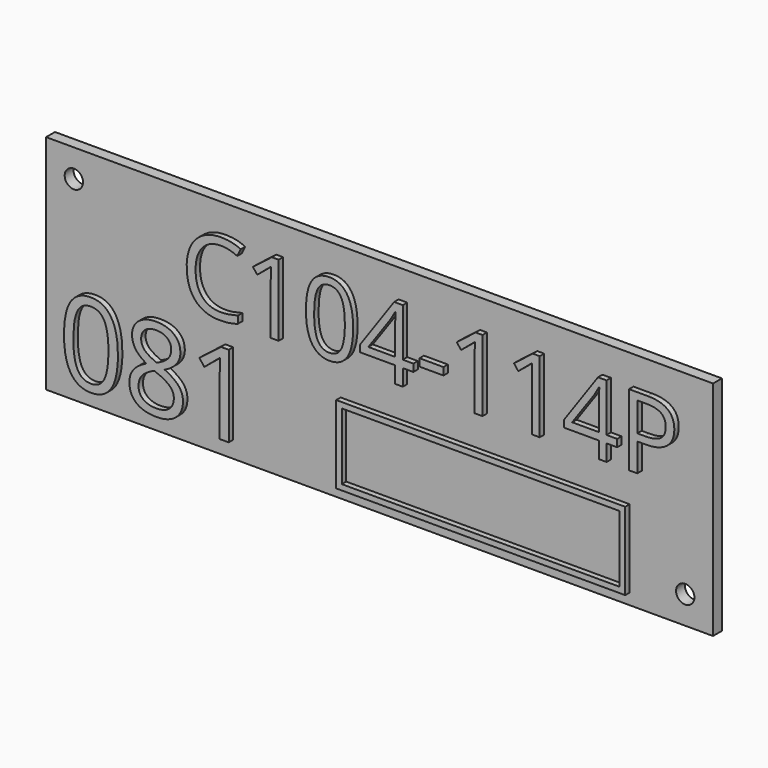
from build123d import *

# Parameters (mm, degrees)
F0_W         = 120
F0_H         = 40
F1_DEPTH     = 2
F3_D         = 3.3
F4_TEXT_SIZE = 18.0050639242
F5_DEPTH     = 1
F6_TEXT_SIZE = 20.5478077656
F7_DEPTH     = 1
F8_W         = 52
F8_H         = 14
F8_W_2       = 49.99999962
F8_H_2       = 11.99999962
F9_DEPTH     = 1


# Not quite as in the source:
# - Text() gives the source's letters only with a copy of the font that has no kerning and outlines rounded to 1/6400 em; it was checked with that copy


with BuildPart() as f1:
    # F0 (on Front) → F1 (new body)
    with BuildSketch(Plane.XZ):
        Rectangle(F0_W, F0_H)
    extrude(amount=F1_DEPTH)

    # F3 (through all)
    with Locations(Plane.XZ.offset(2)):
        with Locations((-55, 15), (55, -15)):
            Hole(F3_D / 2)

    # F4 (on face) → F5 (join)
    with BuildSketch(Plane.XZ.offset(2)):
        with Locations((-35, 2)):
            Text('C104-114P', F4_TEXT_SIZE, font='Open Sans', text_align=(TextAlign.LEFT, TextAlign.BOTTOM))
    extrude(amount=F5_DEPTH)

    # F6 (on face) → F7 (join)
    with BuildSketch(Plane.XZ.offset(2)):
        with Locations((-57, -17)):
            Text('081', F6_TEXT_SIZE, font='Open Sans', text_align=(TextAlign.LEFT, TextAlign.BOTTOM))
    extrude(amount=F7_DEPTH)

    # F8 (on face) → F9 (join)
    with BuildSketch(Plane.XZ.offset(2)):
        with Locations((19, -11)):
            Rectangle(F8_W, F8_H)
        with Locations((19, -11)):
            Rectangle(F8_W_2, F8_H_2, mode=Mode.SUBTRACT)
    extrude(amount=F9_DEPTH)


solid = f1.part
